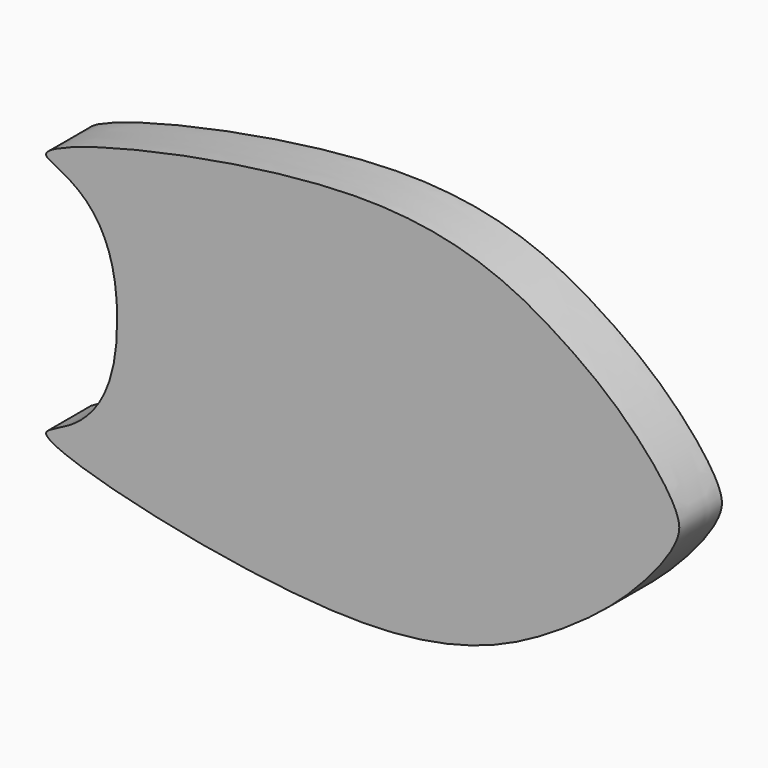
from build123d import *

# Parameters (mm, degrees)
F1_DEPTH = 25.4


# Not quite as in the source:
# - a feature names something its author has since deleted; it is built from what else it names


with BuildPart() as f1:
    # F0 (on Front) → F1 (new body)
    with BuildSketch(Plane.XZ):
        with BuildLine():
            add(Edge.make_bspline(
                [(-115.4564102077, 0), (-115.0665396482, 54.1428744661), (-205.2440837339, 52.4973201914), (13.1909733543, 106.206477706), (92.9880395211, 65.3950430383), (132.5552585521, 34.0234377916), (152.4, 7.4514596081), (152.4, 0)],
                knots=[0, 0, 0, 0, 0.1892861088, 0.4727157898, 0.7011531101, 0.8636916169, 1, 1, 1, 1], degree=3))
            add(Edge.make_bspline(
                [(-115.4564102077, 0), (-115.0665396482, -54.1428744661), (-205.2440837339, -52.4973201914), (13.1909733543, -106.206477706), (92.9880395211, -65.3950430383), (132.5552585521, -34.0234377916), (152.4, -7.4514596081), (152.4, 0)],
                knots=[0, 0, 0, 0, 0.1892861088, 0.4727157898, 0.7011531101, 0.8636916169, 1, 1, 1, 1], degree=3))
        make_face()
    extrude(amount=F1_DEPTH)


solid = f1.part
